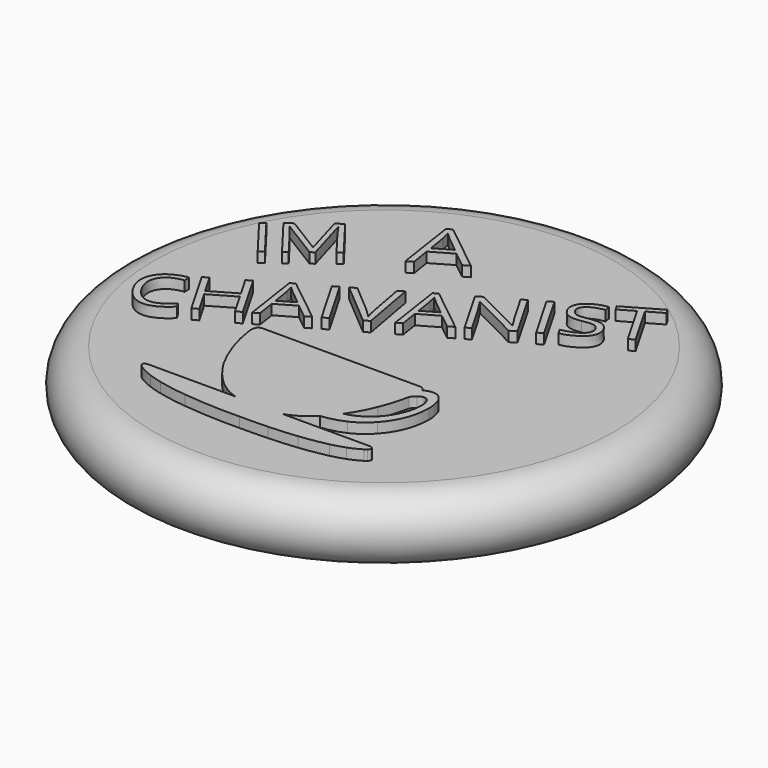
from build123d import *

# Parameters (mm, degrees)
F0_W           = 30.2045792341
F0_H           = 8.6757838726
F4_DEPTH       = 3
F5_TEXT_SIZE   = 8.9257030696
F5_TEXT_SIZE_2 = 10.7108434248
F5_TEXT_SIZE_3 = 9.8182729238
F6_DEPTH       = 3


# Not quite as in the source:
# - ends of sketch curves that miss each other by under 0.0002 mm in the source are joined
# - Text() gives the source's letters only with a copy of the font that has no kerning and outlines rounded to 1/6400 em; it was checked with that copy


with BuildPart() as f1:
    # F0 (on Front) → F1 (revolve)
    with BuildSketch(Plane.XZ):
        with Locations((-15.1022896171, 4.3378919363)):
            Rectangle(F0_W, F0_H)
        with BuildLine():
            ThreePointArc((-30.2045792341, 8.6757838726), (-34.5424711704, 4.3378919363), (-30.2045792341, 0))
            Line((-30.2045792341, 0), (-30.2045792341, 8.6757838726))
        make_face()
    revolve(axis=Axis((0, 0, 4.3378919363), (0, 0, 1)))

    # F3 (on offset) → F4 (join)
    with BuildSketch(Plane.XY.offset(10)):
        with BuildLine():
            ThreePointArc((14.743152502, -20.5270482733), (14.7166592632, -20.3438768195), (14.5758131095, -20.2238100291))
            ThreePointArc((14.5758131095, -20.2238100291), (14.3964399509, -20.1582614009), (14.2060340976, -20.1435127131))
            Line((14.2060340976, -20.1435127131), (2.8549452846, -20.1435110187))
            ThreePointArc((2.8549452846, -20.1435110187), (3.7536447365, -19.7918955578), (4.5917071291, -19.3134127361))
            ThreePointArc((4.5917071291, -19.3134127361), (5.3727269154, -18.7462131817), (6.09045603, -18.1007881932))
            ThreePointArc((6.09045603, -18.1007881932), (7.6156729783, -17.8374930556), (9.0738897209, -17.3186316738))
            ThreePointArc((9.0738897209, -17.3186316738), (10.403176613, -16.5259400173), (11.5525769326, -15.4894852914))
            ThreePointArc((11.5525769326, -15.4894852914), (13.1767604797, -12.8678808553), (13.7443973315, -9.8366137539))
            ThreePointArc((13.7443973315, -9.8366137539), (13.6558738281, -8.8539618418), (13.3923783247, -7.903168424))
            ThreePointArc((13.3923783247, -7.903168424), (13.141760492, -7.4787273431), (12.8055733974, -7.1182584904))
            ThreePointArc((12.8055733974, -7.1182584904), (12.3717359266, -6.8860428934), (11.8854787821, -6.8105893478))
            ThreePointArc((11.8854787821, -6.8105893478), (11.2809691384, -6.9040330672), (10.7328887136, -7.1756428087))
            ThreePointArc((10.7328887136, -7.1756428087), (10.3892002186, -6.7501720734), (9.8564801173, -6.6262505022))
            Line((9.8564801173, -6.6262505022), (-10.6055367215, -6.6262505832))
            ThreePointArc((-10.6055367215, -6.6262505832), (-11.0100535858, -6.7616155906), (-11.248903895, -7.1150380874))
            ThreePointArc((-11.248903895, -7.1150380874), (-11.3314737008, -7.5431509162), (-11.299720517, -7.9779954441))
            ThreePointArc((-11.299720517, -7.9779954441), (-10.4221053603, -11.6710588658), (-8.875212544, -15.1374764723))
            ThreePointArc((-8.875212544, -15.1374764723), (-7.8154409167, -16.7138051098), (-6.5636166028, -18.1423929679))
            ThreePointArc((-6.5636166028, -18.1423929679), (-5.8507811897, -18.7706817008), (-5.0823776957, -19.3296371216))
            ThreePointArc((-5.0823776957, -19.3296371216), (-4.2525413656, -19.7916731306), (-3.3703164957, -20.1435105569))
            Line((-3.3703164957, -20.1435105569), (-14.7184314609, -20.1435110187))
            ThreePointArc((-14.7184314609, -20.1435110187), (-14.9050368026, -20.1620234146), (-15.0830107542, -20.2210986735))
            ThreePointArc((-15.0830107542, -20.2210986735), (-15.2145879337, -20.3453421191), (-15.2568481522, -20.5213051652))
            ThreePointArc((-15.2568481522, -20.5213051652), (-15.1844923413, -20.6956245609), (-15.0526723252, -20.8307026532))
            ThreePointArc((-15.0526723252, -20.8307026532), (-14.9081453734, -20.9556867496), (-14.7515231805, -21.065132907))
            ThreePointArc((-14.7515231805, -21.065132907), (-13.9473606124, -21.5247399819), (-13.0893617475, -21.873673402))
            ThreePointArc((-13.0893617475, -21.873673402), (-12.2094518309, -22.1640523319), (-11.3126510848, -22.3970958074))
            ThreePointArc((-11.3126510848, -22.3970958074), (-9.4961207059, -22.7630035731), (-7.6587596944, -23.0033660322))
            ThreePointArc((-7.6587596944, -23.0033660322), (-3.9629814784, -23.2921557851), (-0.2562316611, -23.3386605031))
            ThreePointArc((-0.2562316611, -23.3386605031), (1.5963720317, -23.3262421686), (3.4483692797, -23.277199672))
            ThreePointArc((3.4483692797, -23.277199672), (5.2982683992, -23.1697572193), (7.14382435, -23.0036252672))
            ThreePointArc((7.14382435, -23.0036252672), (8.9789643737, -22.7498668761), (10.7977828918, -22.397672983))
            ThreePointArc((10.7977828918, -22.397672983), (11.6931620416, -22.1598157094), (12.5745785069, -21.8745283888))
            ThreePointArc((12.5745785069, -21.8745283888), (13.4274598396, -21.512237762), (14.2391013674, -21.0651339675))
            ThreePointArc((14.2391013674, -21.0651339675), (14.3916841827, -20.9552815894), (14.5359697555, -20.834739559))
            ThreePointArc((14.5359697555, -20.834739559), (14.6567639869, -20.6924765799), (14.743152502, -20.5270482733))
        make_face()
        with BuildLine():
            ThreePointArc((11.2896035084, -13.9139501493), (9.6752264231, -15.3945219173), (7.6545687161, -16.2402456103))
            ThreePointArc((7.6545687161, -16.2402456103), (8.6711759867, -14.5891332075), (9.4881962155, -12.8306880419))
            ThreePointArc((9.4881962155, -12.8306880419), (10.1296434807, -11.0007992384), (10.5911626514, -9.1174630569))
            ThreePointArc((10.5911626514, -9.1174630569), (10.8360330219, -8.8035198511), (11.1199539242, -8.5243911135))
            ThreePointArc((11.1199539242, -8.5243911135), (11.4595927355, -8.3225003439), (11.8421683322, -8.2237565996))
            ThreePointArc((11.8421683322, -8.2237565996), (12.0936729001, -8.2697697581), (12.3115524318, -8.4035592202))
            ThreePointArc((12.3115524318, -8.4035592202), (12.4799289094, -8.5977789787), (12.5941720519, -8.8280405118))
            ThreePointArc((12.5941720519, -8.8280405118), (12.735280618, -9.3227785896), (12.7608192795, -9.836611903))
            ThreePointArc((12.7608192795, -9.836611903), (12.6556712771, -10.9327797851), (12.3454986222, -11.9893942937))
            ThreePointArc((12.3454986222, -11.9893942937), (11.8896667706, -12.9912390264), (11.2896035084, -13.9139501493))
        make_face(mode=Mode.SUBTRACT)
    extrude(amount=-F4_DEPTH)

    # F5 (on offset) → F6 (join)
    with BuildSketch(Plane.XY.offset(10)):
        with Locations(Location((-22.2846737385, 5.7838545181), (0, 0, 37.3395242906))):
            Text('IM', F5_TEXT_SIZE, font='Open Sans', text_align=(TextAlign.LEFT, TextAlign.BOTTOM))
        with Locations(Location((-8.4911246, 14.100123945), (0, 0, 30))):
            Text('A', F5_TEXT_SIZE_2, font='Open Sans', text_align=(TextAlign.LEFT, TextAlign.BOTTOM))
        with Locations(Location((-25.2431391637, -11.2927181579), (0, 0, 30))):
            Text('CHAIVANIST', F5_TEXT_SIZE_3, font='Open Sans', text_align=(TextAlign.LEFT, TextAlign.BOTTOM))
    extrude(amount=-F6_DEPTH)


solid = f1.part
